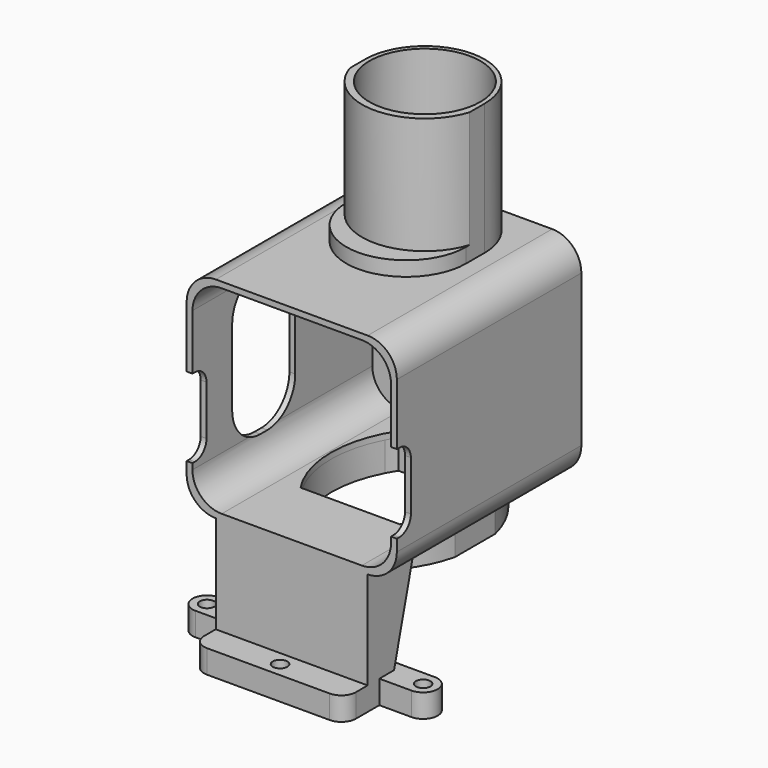
from build123d import *

# Parameters (mm, degrees)
F0_R      = 11.5
F1_DEPTH  = 2
F3_DEPTH  = 77
F5_DEPTH  = 3
F7_DEPTH  = 3
F9_DEPTH  = 5
F11_DEPTH = 3
F12_R     = 19
F13_DEPTH = 8
F14_R     = 19
F15_DEPTH = 40
F16_W     = 52
F16_H     = 3
F17_DEPTH = 38.5
F19_DEPTH = 3
F21_DEPTH = 10
F22_W     = 3
F22_H     = 38.5
F23_DEPTH = 5
F25_R     = 2.5
F25_W     = 47
F25_H     = 2
F26_DEPTH = 5
F27_DEPTH = 1
F29_DEPTH = 75
F30_DEPTH = 2


with BuildPart() as f1:
    # F0 (on Front) → F1 (new body)
    with BuildSketch(Plane.XZ):
        with BuildLine():
            Line((26, 36), (-26, 36))
            ThreePointArc((-26, 36), (-33.0710678119, 33.0710678119), (-36, 26))
            Line((-36, 26), (-36, -26))
            ThreePointArc((-36, -26), (-33.0710678119, -33.0710678119), (-26, -36))
            Line((-26, -36), (26, -36))
            ThreePointArc((26, -36), (33.0710678119, -33.0710678119), (36, -26))
            Line((36, -26), (36, 26))
            ThreePointArc((36, 26), (33.0710678119, 33.0710678119), (26, 36))
        make_face()
        with BuildLine():
            Line((24, -34), (-24, -34))
            ThreePointArc((-24, -34), (-31.0710678119, -31.0710678119), (-34, -24))
            Line((-34, -24), (-34, 24))
            ThreePointArc((-34, 24), (-31.0710678119, 31.0710678119), (-24, 34))
            Line((-24, 34), (24, 34))
            ThreePointArc((24, 34), (31.0710678119, 31.0710678119), (34, 24))
            Line((34, 24), (34, -24))
            ThreePointArc((34, -24), (31.0710678119, -31.0710678119), (24, -34))
        make_face(mode=Mode.SUBTRACT)
        with BuildLine():
            ThreePointArc((-34, -24), (-31.0710678119, -31.0710678119), (-24, -34))
            Line((-24, -34), (24, -34))
            ThreePointArc((24, -34), (31.0710678119, -31.0710678119), (34, -24))
            Line((34, -24), (34, 24))
            ThreePointArc((34, 24), (31.0710678119, 31.0710678119), (24, 34))
            Line((24, 34), (-24, 34))
            ThreePointArc((-24, 34), (-31.0710678119, 31.0710678119), (-34, 24))
            Line((-34, 24), (-34, -24))
        make_face()
        Circle(F0_R, mode=Mode.SUBTRACT)
    extrude(amount=F1_DEPTH)

    # F2 (on face) → F3 (join)
    with BuildSketch(Plane.XZ.offset(2)):
        with BuildLine():
            Line((26, 36), (-26, 36))
            ThreePointArc((-26, 36), (-33.0710678119, 33.0710678119), (-36, 26))
            Line((-36, 26), (-36, -26))
            ThreePointArc((-36, -26), (-33.0710678119, -33.0710678119), (-26, -36))
            Line((-26, -36), (26, -36))
            ThreePointArc((26, -36), (33.0710678119, -33.0710678119), (36, -26))
            Line((36, -26), (36, 26))
            ThreePointArc((36, 26), (33.0710678119, 33.0710678119), (26, 36))
        make_face()
        with BuildLine():
            Line((24, -34), (-24, -34))
            ThreePointArc((-24, -34), (-31.0710678119, -31.0710678119), (-34, -24))
            Line((-34, -24), (-34, 24))
            ThreePointArc((-34, 24), (-31.0710678119, 31.0710678119), (-24, 34))
            Line((-24, 34), (24, 34))
            ThreePointArc((24, 34), (31.0710678119, 31.0710678119), (34, 24))
            Line((34, 24), (34, -24))
            ThreePointArc((34, -24), (31.0710678119, -31.0710678119), (24, -34))
        make_face(mode=Mode.SUBTRACT)
    extrude(amount=F3_DEPTH)

    # F4 (on face) → F5 (cut)
    with BuildSketch(Plane(origin=(-36, 0, 0), x_dir=(0, -1, 0), z_dir=(-1, 0, 0))):
        with BuildLine():
            ThreePointArc((62, 13), (58.4852813742, 21.4852813742), (50, 25))
            Line((50, 25), (47, 25))
            ThreePointArc((47, 25), (38.5147186258, 21.4852813742), (35, 13))
            Line((35, 13), (35, -13))
            ThreePointArc((35, -13), (38.5147186258, -21.4852813742), (47, -25))
            Line((47, -25), (50, -25))
            ThreePointArc((50, -25), (58.4852813742, -21.4852813742), (62, -13))
            Line((62, -13), (62, 13))
        make_face()
    extrude(amount=-F5_DEPTH, mode=Mode.SUBTRACT)

    # F6 (on face) → F7 (cut)
    with BuildSketch(Plane.XY.offset(36)):
        with BuildLine():
            Line((19, -30), (19, -22))
            ThreePointArc((19, -22), (0, -3), (-19, -22))
            Line((-19, -22), (-19, -30))
            ThreePointArc((-19, -30), (0, -49), (19, -30))
        make_face()
    extrude(amount=-F7_DEPTH, mode=Mode.SUBTRACT)

    # F8 (on face) → F9 (join)
    with BuildSketch(Plane.XY.offset(36)):
        with BuildLine():
            Line((-20.5, -22), (-20.5, -30))
            ThreePointArc((-20.5, -30), (0, -50.5), (20.5, -30))
            Line((20.5, -30), (20.5, -22))
            ThreePointArc((20.5, -22), (0, -1.5), (-20.5, -22))
        make_face()
        with BuildLine():
            ThreePointArc((-19, -22), (0, -3), (19, -22))
            Line((19, -22), (19, -22.3025978408))
            Line((19, -22.3025978408), (19, -29.6974021592))
            Line((19, -29.6974021592), (19, -30))
            ThreePointArc((19, -30), (0, -49), (-19, -30))
            Line((-19, -30), (-19, -22))
        make_face(mode=Mode.SUBTRACT)
        with BuildLine():
            Line((19, -22.3025978408), (19, -22))
            ThreePointArc((19, -22), (0, -3), (-19, -22))
            Line((-19, -22), (-19, -30))
            ThreePointArc((-19, -30), (0, -49), (19, -30))
            Line((19, -30), (19, -29.6974021592))
            Line((19, -29.6974021592), (19, -22.3025978408))
        make_face()
    extrude(amount=F9_DEPTH)

    # F10 (on face) → F11 (join)
    with BuildSketch(Plane.XY.offset(36)):
        with BuildLine():
            Line((20.5, -30), (20.5, -22))
            ThreePointArc((20.5, -22), (0, -1.5), (-20.5, -22))
            Line((-20.5, -22), (-20.5, -30))
            ThreePointArc((-20.5, -30), (0, -50.5), (20.5, -30))
        make_face()
    extrude(amount=F11_DEPTH)

    # F12 (on face) → F13 (cut)
    with BuildSketch(Plane.XY.offset(41)):
        with Locations((0, -22)):
            Circle(F12_R)
    extrude(amount=-F13_DEPTH, mode=Mode.SUBTRACT)

    # F14 (on face) → F15 (join)
    with BuildSketch(Plane.XY.offset(41)):
        with BuildLine():
            Line((-20.5, -22), (-20.5, -28.4807406984))
            ThreePointArc((-20.5, -28.4807406984), (0, -43.5), (20.5, -28.4807406984))
            Line((20.5, -28.4807406984), (20.5, -22))
            ThreePointArc((20.5, -22), (0, -1.5), (-20.5, -22))
        make_face()
        with Locations((0, -22)):
            Circle(F14_R, mode=Mode.SUBTRACT)
    extrude(amount=F15_DEPTH)

    # F16 (on face) → F17 (join)
    with BuildSketch(Plane(origin=(0, 0, -36), x_dir=(1, 0, 0), z_dir=(0, 0, -1))):
        with Locations((0, 77.5)):
            Rectangle(F16_W, F16_H)
    extrude(amount=F17_DEPTH)

    # F18 (on face) → F19 (cut)
    with BuildSketch(Plane(origin=(0, 0, -36), x_dir=(1, 0, 0), z_dir=(0, 0, -1))):
        with BuildLine():
            Line((-17, 12), (17, 12))
            ThreePointArc((17, 12), (23.3298247558, 33), (17, 54))
            Line((17, 54), (-17, 54))
            ThreePointArc((-17, 54), (-23.3298247558, 33), (-17, 12))
        make_face()
    extrude(amount=-F19_DEPTH, mode=Mode.SUBTRACT)

    # F20 (on face) → F21 (join)
    with BuildSketch(Plane(origin=(0, 0, -36), x_dir=(1, 0, 0), z_dir=(0, 0, -1))):
        with BuildLine():
            ThreePointArc((19, 50.6158820109), (23.3298247558, 33), (19, 15.3841179891))
            Line((19, 15.3841179891), (19, 10))
            ThreePointArc((19, 10), (23.2866263695, 16.8090036252), (26, 24.3836521016))
            Line((26, 24.3836521016), (26, 41.6163478984))
            ThreePointArc((26, 41.6163478984), (23.2866263695, 49.1909963748), (19, 56))
            Line((19, 56), (19, 50.6158820109))
        make_face()
        with BuildLine():
            Line((-19, 56), (-19, 50.6158820109))
            ThreePointArc((-19, 50.6158820109), (-18.0437883513, 52.3338197434), (-17, 54))
            Line((-17, 54), (17, 54))
            ThreePointArc((17, 54), (18.0437883513, 52.3338197434), (19, 50.6158820109))
            Line((19, 50.6158820109), (19, 56))
            Line((19, 56), (-19, 56))
        make_face()
        with BuildLine():
            Line((-19, 10), (-19, 15.3841179891))
            ThreePointArc((-19, 15.3841179891), (-23.3298247558, 33), (-19, 50.6158820109))
            Line((-19, 50.6158820109), (-19, 56))
            ThreePointArc((-19, 56), (-23.2866263695, 49.1909963748), (-26, 41.6163478984))
            Line((-26, 41.6163478984), (-26, 24.3836521016))
            ThreePointArc((-26, 24.3836521016), (-23.2866263695, 16.8090036252), (-19, 10))
        make_face()
        with BuildLine():
            Line((17, 12), (-17, 12))
            ThreePointArc((-17, 12), (-18.0437883513, 13.6661802566), (-19, 15.3841179891))
            Line((-19, 15.3841179891), (-19, 10))
            Line((-19, 10), (19, 10))
            Line((19, 10), (19, 15.3841179891))
            ThreePointArc((19, 15.3841179891), (18.0437883513, 13.6661802566), (17, 12))
        make_face()
    extrude(amount=F21_DEPTH)

    # F22 (on face) → F23 (join)
    with BuildSketch(Plane.YZ.offset(26)):
        Polygon((-76, -36), (-76, -74.5), (-69, -74.5), (-59, -36), align=None)
        with Locations((-77.5, -55.25)):
            Rectangle(F22_W, F22_H)
    extrude(amount=-F23_DEPTH)

    # F25 (on face) → F26 (join)
    with BuildSketch(Plane(origin=(0, 0, -74.5), x_dir=(1, 0, 0), z_dir=(0, 0, -1))):
        with BuildLine():
            Line((37, 74), (26, 74))
            Line((26, 74), (21, 74))
            Line((21, 74), (-26, 74))
            Line((-26, 74), (-37, 74))
            ThreePointArc((-37, 74), (-42, 69), (-37, 64))
            Line((-37, 64), (37, 64))
            ThreePointArc((37, 64), (42, 69), (37, 74))
        make_face()
        with Locations((-37, 69)):
            Circle(F25_R, mode=Mode.SUBTRACT)
        with Locations((0, 69)):
            Circle(F25_R, mode=Mode.SUBTRACT)
        with Locations((37, 69)):
            Circle(F25_R, mode=Mode.SUBTRACT)
        Polygon((26, 79), (-26, 79), (-26, 76), (21, 76), (21, 74), (26, 74), align=None)
        with Locations((-2.5, 75)):
            Rectangle(F25_W, F25_H)
        with BuildLine():
            Line((-26.0336585343, 79), (-26, 79))
            Line((-26, 79), (26, 79))
            Line((26, 79), (26, 84))
            ThreePointArc((26, 84), (24.5355339059, 87.5355339059), (21, 89))
            Line((21, 89), (-21.0336585343, 89))
            ThreePointArc((-21.0336585343, 89), (-24.5691924402, 87.5355339059), (-26.0336585343, 84))
            Line((-26.0336585343, 84), (-26.0336585343, 79))
        make_face()
        with Locations((0, 84)):
            Circle(F25_R, mode=Mode.SUBTRACT)
    extrude(amount=-F26_DEPTH)

    # F27 (add): faces of the model
    f27_faces = [f1.faces().sort_by_distance(p)[0] for p in [
        (23.5, -77.5, -74.5),
        (-2.5, -77.5, -74.5),
        (23.5, -72.5, -74.5),
        (-26.0168292671, -79.5298586246, -74.5),
        (-41.1514718626, -69, -74.5),
    ]]
    extrude(f27_faces, amount=F27_DEPTH)

    # F28 (on face) → F29 (cut)
    with BuildSketch(Plane.YZ.offset(36)):
        with BuildLine():
            Line((-78, 5), (-79, 5))
            Line((-79, 5), (-79, -22))
            Line((-79, -22), (-78, -22))
            ThreePointArc((-78, -22), (-74.4644660941, -20.5355339059), (-73, -17))
            Line((-73, -17), (-73, 0))
            ThreePointArc((-73, 0), (-74.4644660941, 3.5355339059), (-78, 5))
        make_face()
    extrude(amount=-F29_DEPTH, mode=Mode.SUBTRACT)

    # F30 (add): a face of the model
    f30_faces = [f1.faces().sort_by_distance(p)[0] for p in [
        (-0.0056811519, -75.1326620312, -75.5),
    ]]
    extrude(f30_faces, amount=F30_DEPTH)


solid = f1.part
